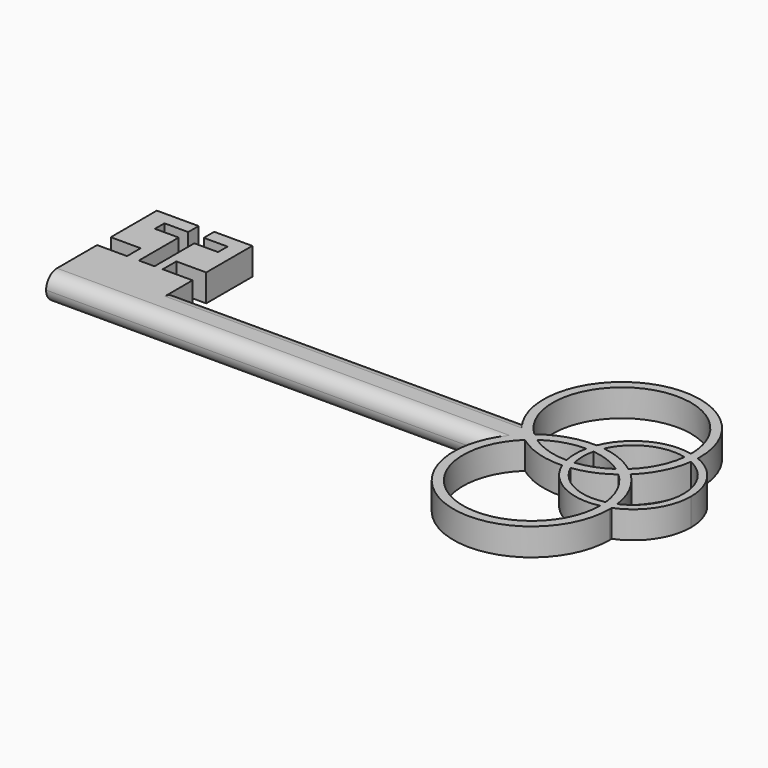
from build123d import *

# Parameters (mm, degrees)
F1_DEPTH = 5
F2_R     = 2.49999
F3_W     = 5.486164242
F3_H     = 3.1326031312
F3_W_2   = 5.482269451
F3_W_3   = 2.8602015227
F3_H_2   = 9.1254087165
F3_H_3   = 2.179203555
F3_H_4   = 2.3905187845
F3_W_4   = 4.3584052473
F3_W_5   = 4.3584033847
F4_DEPTH = 25


# Not quite as in the source:
# - a fillet or chamfer is up to 0.001 mm smaller than in the source, because OpenCascade refuses the exact size


with BuildPart() as f1:
    # F0 (on Top) → F1 (new body)
    with BuildSketch(Plane.XY):
        with BuildLine():
            ThreePointArc((43.1041480843, -1.140358212), (41.4640780002, 0.7201286462), (40.168760519, 2.8351685639))
            Line((40.168760519, 2.8351685639), (-23.6701387912, 2.8351685639))
            Line((-23.6701387912, 2.8351685639), (-23.6701387912, 20.3415267169))
            Line((-23.6701387912, 20.3415267169), (-41.1761775613, 20.3415267169))
            Line((-41.1761775613, 20.3415267169), (-41.1761775613, 2.8351685639))
            Line((-41.1761775613, 2.8351685639), (-41.1761775613, -5.0545609556))
            Line((-41.1761775613, -5.0545609556), (40.2184031878, -5.0545609556))
            ThreePointArc((40.2184031878, -5.0545609556), (41.4937778577, -2.9739718927), (43.1041480843, -1.140358212))
        make_face()
        with BuildLine():
            ThreePointArc((67.3555774067, 8.7261943334), (67.3626426338, 8.9861285841), (67.3649979671, 9.246148169))
            ThreePointArc((67.3649979671, 9.246148169), (49.7178994981, 23.2169748342), (40.168760519, 2.8351685639))
            ThreePointArc((40.168760519, 2.8351685639), (41.4640780002, 0.7201286462), (43.1041480843, -1.140358212))
            ThreePointArc((43.1041480843, -1.140358212), (43.7292665999, -0.5749391558), (44.3865925628, -0.0473081805))
            ThreePointArc((44.3865925628, -0.0473081805), (47.9413125892, 20.8671965928), (65.6900889224, 9.2468057623))
            ThreePointArc((65.6900889224, 9.2468057623), (66.5335502723, 9.0207851567), (67.3555774067, 8.7261943334))
        make_face()
        with BuildLine():
            ThreePointArc((44.4356579567, -2.2642557619), (43.7528332621, -1.7225299618), (43.1041480843, -1.140358212))
            ThreePointArc((43.1041480843, -1.140358212), (41.4937778577, -2.9739718927), (40.2184031878, -5.0545609556))
            ThreePointArc((40.2184031878, -5.0545609556), (49.7174675435, -25.3901824255), (67.3204571559, -11.4652235061))
            ThreePointArc((67.3204571559, -11.4652235061), (67.3182526979, -11.2140597341), (67.3116400033, -10.96297335))
            ThreePointArc((67.3116400033, -10.96297335), (66.4614410979, -11.2621198468), (65.5889276735, -11.4880559652))
            ThreePointArc((65.5889276735, -11.4880559652), (47.9839421141, -22.9945229972), (44.4356579567, -2.2642557619))
        make_face()
        with BuildLine():
            ThreePointArc((73.9806472497, -1.1095376685), (72.169922865, 4.8199052741), (67.3555774067, 8.7261943334))
            ThreePointArc((67.3555774067, 8.7261943334), (67.3117311725, 8.010705268), (67.2322189831, 7.2982974448))
            ThreePointArc((67.2322189831, 7.2982974448), (71.1579723309, 3.8836422981), (72.6206968225, -1.1095376685))
            ThreePointArc((72.6206968225, -1.1095376685), (71.1453970138, -6.1222851765), (67.1899029185, -9.5366978003))
            ThreePointArc((67.1899029185, -9.5366978003), (67.2686178092, -10.2483123334), (67.3116400033, -10.96297335))
            ThreePointArc((67.3116400033, -10.96297335), (72.1566691186, -7.0586101253), (73.9806472497, -1.1095376685))
        make_face()
        with BuildLine():
            ThreePointArc((54.9590998914, -4.9748227507), (54.2466920753, -5.0543350042), (53.5312030139, -5.0981813027))
            ThreePointArc((53.5312030139, -5.0981813027), (58.3970374227, -10.4877579943), (65.5889276735, -11.4880559652))
            ThreePointArc((65.5889276735, -11.4880559652), (65.5889432165, -11.4766397403), (65.5889483975, -11.4652235061))
            ThreePointArc((65.5889483975, -11.4652235061), (65.5706384672, -10.7868000494), (65.5157619854, -10.1103518165))
            ThreePointArc((65.5157619854, -10.1103518165), (59.3188229712, -9.4308900821), (54.9590998914, -4.9748227507))
        make_face()
        with BuildLine():
            ThreePointArc((54.3661207024, 1.0392904692), (53.6782725799, 1.094777615), (52.9884165603, 1.1124562812))
            ThreePointArc((52.9884165603, 1.1124562812), (52.7533483797, -1.1613192361), (53.0105914352, -3.4326928652))
            ThreePointArc((53.0105914352, -3.4326928652), (53.7015001008, -3.4138898359), (54.3903575498, -3.3574650805))
            ThreePointArc((54.3903575498, -3.3574650805), (54.1133130855, -1.1605476943), (54.3661207024, 1.0392904692))
        make_face()
        with BuildLine():
            ThreePointArc((65.6900889395, 9.246148169), (65.6900889352, 9.2464769657), (65.6900889224, 9.2468057623))
            ThreePointArc((65.6900889224, 9.2468057623), (58.421880956, 8.2818061592), (53.5134993303, 2.8351685639))
            ThreePointArc((53.5134993303, 2.8351685639), (54.2281603431, 2.7921463054), (54.9397748692, 2.7134313507))
            ThreePointArc((54.9397748692, 2.7134313507), (59.3437953002, 7.2239168329), (65.6148612618, 7.867039641))
            ThreePointArc((65.6148612618, 7.867039641), (65.6712680509, 8.5555687863), (65.6900889395, 9.246148169))
        make_face()
        with BuildLine():
            ThreePointArc((60.2384014175, -1.1712057304), (60.9570485035, -0.6339967178), (61.6359032137, -0.0473081805))
            ThreePointArc((61.6359032137, -0.0473081805), (58.4654054664, 1.7637460297), (54.9397748692, 2.7134313507))
            ThreePointArc((54.9397748692, 2.7134313507), (54.6128353821, 1.8901056598), (54.3661207024, 1.0392904692))
            ThreePointArc((54.3661207024, 1.0392904692), (57.4423163149, 0.3061053356), (60.2384014175, -1.1712057304))
        make_face()
        with BuildLine():
            ThreePointArc((53.5134993303, 2.8351685639), (48.7018941946, 2.1796634707), (44.3865925628, -0.0473081805))
            ThreePointArc((44.3865925628, -0.0473081805), (45.0654472729, -0.6339967178), (45.7840943589, -1.1712057304))
            ThreePointArc((45.7840943589, -1.1712057304), (49.2106758058, 0.5245305343), (52.9884165603, 1.1124562812))
            ThreePointArc((52.9884165603, 1.1124562812), (53.2143527571, 1.9849696853), (53.5134993303, 2.8351685639))
        make_face()
        with BuildLine():
            ThreePointArc((44.3865925628, -0.0473081805), (43.7292665999, -0.5749391558), (43.1041480843, -1.140358212))
            ThreePointArc((43.1041480843, -1.140358212), (43.7528332621, -1.7225299618), (44.4356579567, -2.2642557619))
            ThreePointArc((44.4356579567, -2.2642557619), (45.0909975882, -1.6944412812), (45.7840943589, -1.1712057304))
            ThreePointArc((45.7840943589, -1.1712057304), (45.0654472729, -0.6339967178), (44.3865925628, -0.0473081805))
        make_face()
        with BuildLine():
            ThreePointArc((45.7840943589, -1.1712057304), (45.0909975882, -1.6944412812), (44.4356579567, -2.2642557619))
            ThreePointArc((44.4356579567, -2.2642557619), (48.7414590733, -4.4578309904), (53.5312030139, -5.0981813027))
            ThreePointArc((53.5312030139, -5.0981813027), (53.2366121166, -4.2761541948), (53.0105914352, -3.4326928652))
            ThreePointArc((53.0105914352, -3.4326928652), (49.2245751666, -2.854022082), (45.7840943589, -1.1712057304))
        make_face()
        with BuildLine():
            ThreePointArc((53.0105914352, -3.4326928652), (53.2366121166, -4.2761541948), (53.5312030139, -5.0981813027))
            ThreePointArc((53.5312030139, -5.0981813027), (54.2466920753, -5.0543350042), (54.9590998914, -4.9748227507))
            ThreePointArc((54.9590998914, -4.9748227507), (54.6371920778, -4.1793436416), (54.3903575498, -3.3574650805))
            ThreePointArc((54.3903575498, -3.3574650805), (53.7015001008, -3.4138898359), (53.0105914352, -3.4326928652))
        make_face()
        with BuildLine():
            ThreePointArc((54.9397748692, 2.7134313507), (54.2281603431, 2.7921463054), (53.5134993303, 2.8351685639))
            ThreePointArc((53.5134993303, 2.8351685639), (53.2143527571, 1.9849696853), (52.9884165603, 1.1124562812))
            ThreePointArc((52.9884165603, 1.1124562812), (53.6782725799, 1.094777615), (54.3661207024, 1.0392904692))
            ThreePointArc((54.3661207024, 1.0392904692), (54.6128353821, 1.8901056598), (54.9397748692, 2.7134313507))
        make_face()
        with BuildLine():
            ThreePointArc((54.9590998914, -4.9748227507), (58.4447091137, -4.0394696351), (61.5868378197, -2.2642557619))
            ThreePointArc((61.5868378197, -2.2642557619), (60.9314981882, -1.6944412812), (60.2384014175, -1.1712057304))
            ThreePointArc((60.2384014175, -1.1712057304), (57.4510535162, -2.6299259461), (54.3903575498, -3.3574650805))
            ThreePointArc((54.3903575498, -3.3574650805), (54.6371920778, -4.1793436416), (54.9590998914, -4.9748227507))
        make_face()
        with BuildLine():
            ThreePointArc((61.5868378197, -2.2642557619), (62.2696625143, -1.7225299618), (62.9183476921, -1.140358212))
            ThreePointArc((62.9183476921, -1.140358212), (62.2932291765, -0.5749391558), (61.6359032137, -0.0473081805))
            ThreePointArc((61.6359032137, -0.0473081805), (60.9570485035, -0.6339967178), (60.2384014175, -1.1712057304))
            ThreePointArc((60.2384014175, -1.1712057304), (60.9314981882, -1.6944412812), (61.5868378197, -2.2642557619))
        make_face()
        with BuildLine():
            ThreePointArc((62.9183476921, -1.140358212), (65.7918456304, 2.7126603808), (67.2322189831, 7.2982974448))
            ThreePointArc((67.2322189831, 7.2982974448), (66.4367398451, 7.6202051868), (65.6148612618, 7.867039641))
            ThreePointArc((65.6148612618, 7.867039641), (64.3390487935, 3.5510680946), (61.6359032137, -0.0473081805))
            ThreePointArc((61.6359032137, -0.0473081805), (62.2932291765, -0.5749391558), (62.9183476921, -1.140358212))
        make_face()
        with BuildLine():
            ThreePointArc((67.2322189831, 7.2982974448), (67.3117311725, 8.010705268), (67.3555774067, 8.7261943334))
            ThreePointArc((67.3555774067, 8.7261943334), (66.5335502723, 9.0207851567), (65.6900889224, 9.2468057623))
            ThreePointArc((65.6900889224, 9.2468057623), (65.6900889352, 9.2464769657), (65.6900889395, 9.246148169))
            ThreePointArc((65.6900889395, 9.246148169), (65.6712680509, 8.5555687863), (65.6148612618, 7.867039641))
            ThreePointArc((65.6148612618, 7.867039641), (66.4367398451, 7.6202051868), (67.2322189831, 7.2982974448))
        make_face()
        with BuildLine():
            ThreePointArc((67.1899029185, -9.5366978003), (65.7648954489, -4.9769306827), (62.9183476921, -1.140358212))
            ThreePointArc((62.9183476921, -1.140358212), (62.2696625143, -1.7225299618), (61.5868378197, -2.2642557619))
            ThreePointArc((61.5868378197, -2.2642557619), (64.2577141016, -5.8335676384), (65.5157619854, -10.1103518165))
            ThreePointArc((65.5157619854, -10.1103518165), (66.3665771981, -9.8636372133), (67.1899029185, -9.5366978003))
        make_face()
        with BuildLine():
            ThreePointArc((65.5889276735, -11.4880559652), (66.4614410979, -11.2621198468), (67.3116400033, -10.96297335))
            ThreePointArc((67.3116400033, -10.96297335), (67.2686178092, -10.2483123334), (67.1899029185, -9.5366978003))
            ThreePointArc((67.1899029185, -9.5366978003), (66.3665771981, -9.8636372133), (65.5157619854, -10.1103518165))
            ThreePointArc((65.5157619854, -10.1103518165), (65.5706384672, -10.7868000494), (65.5889483975, -11.4652235061))
            ThreePointArc((65.5889483975, -11.4652235061), (65.5889432165, -11.4766397403), (65.5889276735, -11.4880559652))
        make_face()
    extrude(amount=F1_DEPTH)

    # F2 (radius 2.5 in the source; OpenCascade refuses exactly that, so slightly less here)
    f2_edges = [f1.edges().sort_by_distance(p)[0] for p in [
        (-0.478887, -5.054561, 5),
        (-0.478887, -5.054561, 0),
        (8.249311, 2.835169, 5),
        (8.249311, 2.835169, 0),
    ]]
    fillet(f2_edges, radius=F2_R)

    # F3 (on face) → F4 (cut)
    with BuildSketch(Plane(origin=(0, 0, 0), x_dir=(1, 0, 0), z_dir=(0, 0, -1))):
        with Locations((-38.4330954403, -8.2126972266)):
            Rectangle(F3_W, F3_H)
        with Locations((-26.4112735167, -8.2126972266)):
            Rectangle(F3_W_2, F3_H)
        with Locations((-32.0807108656, -11.2091000192)):
            Rectangle(F3_W_3, F3_H_2)
        with Locations((-32.0807108656, -16.8614061549)):
            Rectangle(F3_W_3, F3_H_3)
        with Locations((-32.0807108656, -19.1462673247)):
            Rectangle(F3_W_3, F3_H_4)
        with Locations((-28.4714074805, -16.8614061549)):
            Rectangle(F3_W_4, F3_H_3)
        with Locations((-35.6900133193, -16.8614061549)):
            Rectangle(F3_W_5, F3_H_3)
    extrude(amount=-F4_DEPTH, mode=Mode.SUBTRACT)


solid = f1.part
